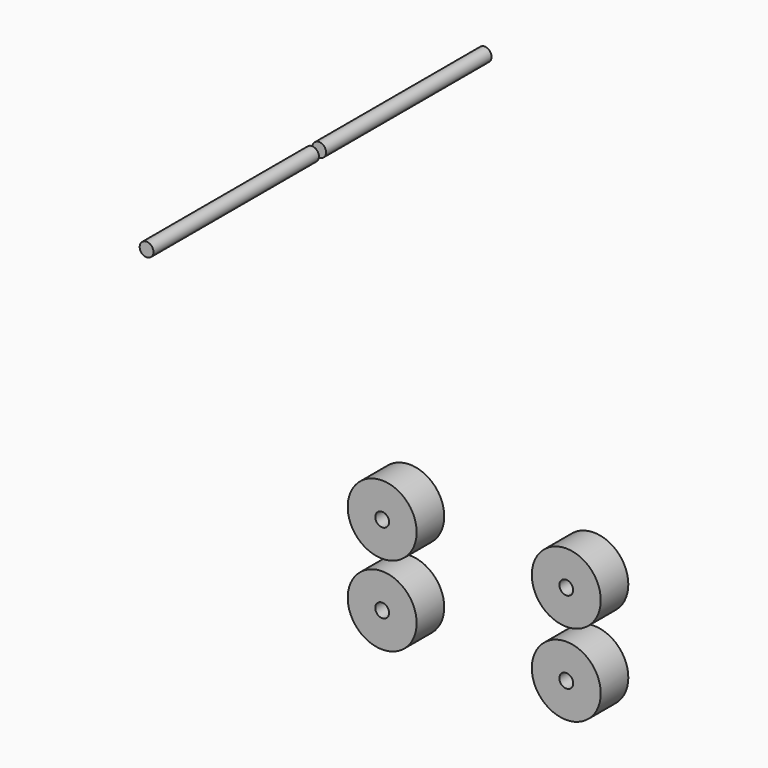
from build123d import *

# Parameters (mm, degrees)
F0_R     = 12.7
F0_R_2   = 2.54
F1_DEPTH = 12.7
F2_DEPTH = 12.7
F6_R     = 2.54
F7_DEPTH = 76.2


# Not quite as in the source:
# - a feature names something its author has since deleted; it is built from what else it names


with BuildPart() as f1:
    # F0 (on Front) → F1 (new body)
    with BuildSketch(Plane.XZ):
        with Locations((-35.070437938, -31.5513052046)):
            Circle(F0_R)
        with Locations((-35.070437938, -31.5513052046)):
            Circle(F0_R_2, mode=Mode.SUBTRACT)
    extrude(amount=F1_DEPTH)

    # F0 (on Front) → F2 (join)
    with BuildSketch(Plane.XZ):
        with Locations((-35.070437938, -31.5513052046)):
            Circle(F0_R)
        with Locations((-35.070437938, -31.5513052046)):
            Circle(F0_R_2, mode=Mode.SUBTRACT)
    extrude(amount=F2_DEPTH)


with BuildPart() as f3_1:
    # F3: copy of F1
    add(f1.part.moved(Location((67.818, 0, 0))))


with BuildPart() as f4_1:
    # F4: copy of F3_1
    add(f3_1.part.moved(Location((0, 0, -30.226))))


with BuildPart() as f5_1:
    # F5: copy of F1
    add(f1.part.moved(Location((0, 0, -29.464))))


with BuildPart() as f7:
    # F6 (on Front) → F7 (new body)
    with BuildSketch(Plane.XZ):
        with Locations((-71.0687860847, 70.1470151544)):
            Circle(F6_R)
    extrude(amount=F7_DEPTH)


with BuildPart() as f8_1:
    # F8: copy of F7
    add(f7.part.moved(Location((0, 79.502, 0))))


solid = Compound([f1.part, f3_1.part, f4_1.part, f5_1.part, f7.part, f8_1.part])
